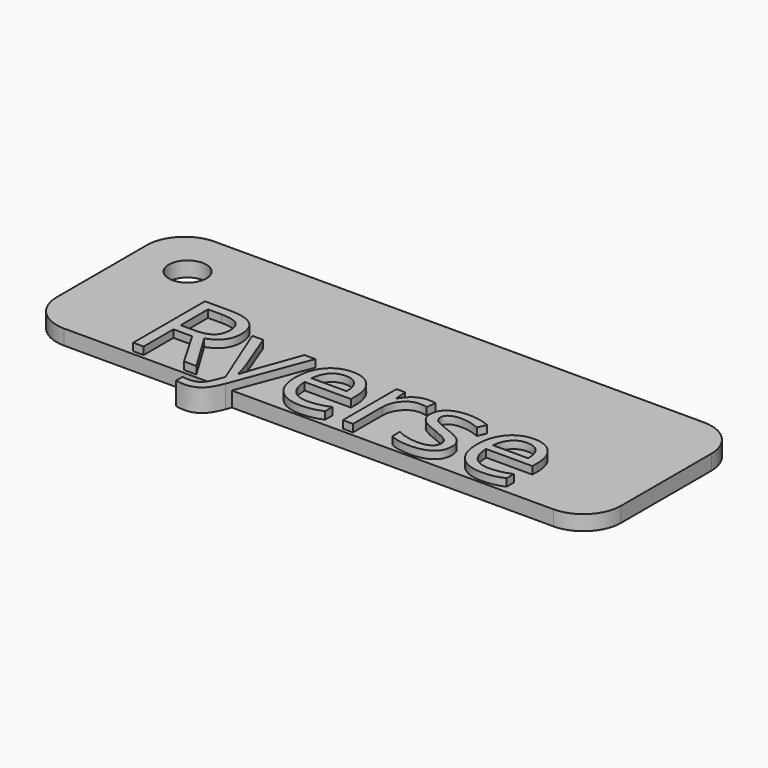
from build123d import *

# Parameters (mm, degrees)
F1_DEPTH     = 2
F3_D         = 5
F4_TEXT_SIZE = 16.666668105
F5_DEPTH     = 3


# Not quite as in the source:
# - Text() gives the source's letters only with a copy of the font that has no kerning and outlines rounded to 1/6400 em; it was checked with that copy


with BuildPart() as f1:
    # F0 (on Top) → F1 (new body)
    with BuildSketch(Plane.XY):
        with BuildLine():
            Line((32.5, 12.5), (-32.5, 12.5))
            ThreePointArc((-32.5, 12.5), (-36.0355339059, 11.0355339059), (-37.5, 7.5))
            Line((-37.5, 7.5), (-37.5, -7.5))
            ThreePointArc((-37.5, -7.5), (-36.0355339059, -11.0355339059), (-32.5, -12.5))
            Line((-32.5, -12.5), (32.5, -12.5))
            ThreePointArc((32.5, -12.5), (36.0355339059, -11.0355339059), (37.5, -7.5))
            Line((37.5, -7.5), (37.5, 7.5))
            ThreePointArc((37.5, 7.5), (36.0355339059, 11.0355339059), (32.5, 12.5))
        make_face()
    extrude(amount=F1_DEPTH)

    # F3 (through all)
    with Locations(Plane(origin=(0, 0, 0), x_dir=(1, 0, 0), z_dir=(0, 0, -1))):
        with Locations((-30.5, -5.5)):
            Hole(F3_D / 2)

    # F4 (on Top) → F5 (join)
    with BuildSketch(Plane.XY):
        with Locations((-25.3499988467, -12.0000010356)):
            Text('Ryerse', F4_TEXT_SIZE, font='Open Sans', text_align=(TextAlign.LEFT, TextAlign.BOTTOM))
    extrude(amount=F5_DEPTH)


solid = f1.part
